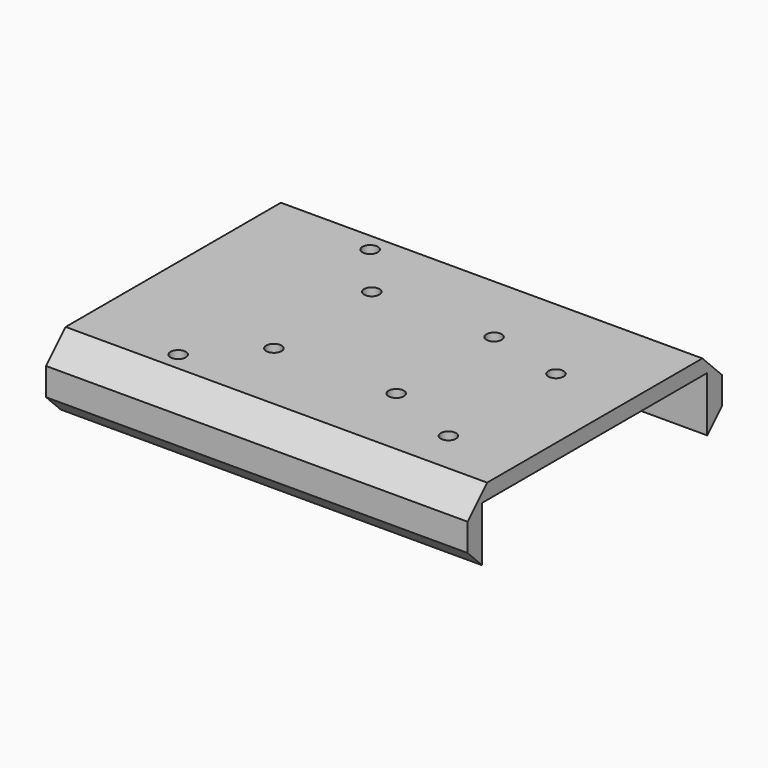
from build123d import *

# Parameters (mm, degrees)
F0_W        = 87.5494211584
F0_H        = 66.04
F0_R        = 1.5875
F1_DEPTH    = 3.175
F2_R        = 3.175
F2_R_2      = 1.5875
F3_DEPTH    = 3.175
F4_DEPTH    = 25.4
F5_W        = 87.5494211584
F5_H        = 3.81
F6_DEPTH    = 12.7
F7_T1_DEPTH = 113.6777203162


# Not quite as in the source:
# - a fillet or chamfer that OpenCascade refuses, or shapes differently, is made with other operations: its cross-section is extruded or revolved along the edge and cut away or added


with BuildPart() as f1:
    # F0 (on Top) → F1 (new body)
    with BuildSketch(Plane.XY):
        with Locations((22.1847105792, -24.13)):
            Rectangle(F0_W, F0_H)
        with Locations((-1.27, -48.26)):
            Circle(F0_R, mode=Mode.SUBTRACT)
        with Locations((50.8, -43.18)):
            Circle(F0_R, mode=Mode.SUBTRACT)
        Circle(F0_R, mode=Mode.SUBTRACT)
        with Locations((50.8, -15.24)):
            Circle(F0_R, mode=Mode.SUBTRACT)
    extrude(amount=F1_DEPTH)

    # F2 (on face) → F3 (join)
    with BuildSketch(Plane(origin=(0, 0, 0), x_dir=(1, 0, 0), z_dir=(0, 0, -1))):
        with Locations((9.4847105792, 11.43)):
            Circle(F2_R)
        with Locations((9.4847105792, 11.43)):
            Circle(F2_R_2, mode=Mode.SUBTRACT)
        with Locations((9.4847105792, 36.83)):
            Circle(F2_R)
        with Locations((9.4847105792, 36.83)):
            Circle(F2_R_2, mode=Mode.SUBTRACT)
        with Locations((34.8847105792, 36.83)):
            Circle(F2_R)
        with Locations((34.8847105792, 36.83)):
            Circle(F2_R_2, mode=Mode.SUBTRACT)
        with Locations((34.8847105792, 11.43)):
            Circle(F2_R)
        with Locations((34.8847105792, 11.43)):
            Circle(F2_R_2, mode=Mode.SUBTRACT)
    extrude(amount=F3_DEPTH)

    # F4 (cut): faces of the model
    f4_faces = [f1.faces().sort_by_distance(p)[0] for p in [
        (9.4847105792, -11.43, 0),
        (9.4847105792, -36.83, 0),
        (34.8847105792, -36.83, 0),
        (34.8847105792, -11.43, 0),
    ]]
    extrude(f4_faces, amount=-F4_DEPTH, mode=Mode.SUBTRACT)

    # F5 (on face) → F6 (join)
    with BuildSketch(Plane(origin=(0, 0, 0), x_dir=(1, 0, 0), z_dir=(0, 0, -1))):
        with Locations((22.1847105792, -6.985)):
            Rectangle(F5_W, F5_H)
        with Locations((22.1847105792, 55.245)):
            Rectangle(F5_W, F5_H)
    extrude(amount=F6_DEPTH)

    # F7: chamfer of 5.08 on 4 edges, made by hand

    # F7_s2 → F7_t1 (cut)
    with BuildSketch(Plane.YZ.offset(-34.6541495789)):
        Polygon((8.89, -1.905), (3.81, 3.175), (8.89, 3.175), align=None)
        Polygon((-52.07, 3.175), (-57.15, -1.905), (-57.15, 3.175), align=None)
        Polygon((3.81, -12.7), (8.89, -7.62), (8.89, -12.7), align=None)
        Polygon((-52.07, -12.7), (-57.15, -7.62), (-57.15, -12.7), align=None)
    extrude(amount=F7_T1_DEPTH, mode=Mode.SUBTRACT)


solid = f1.part
